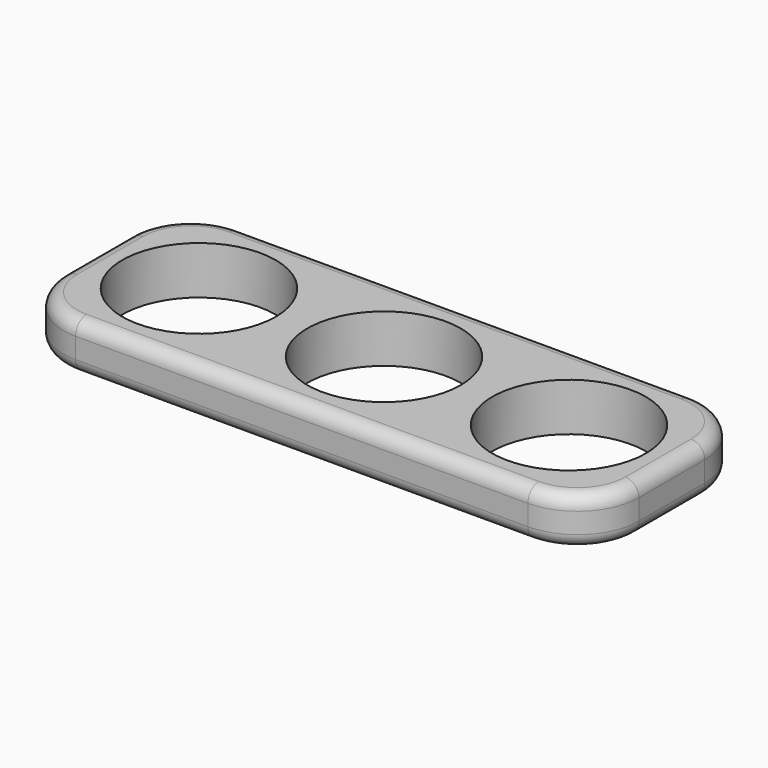
from build123d import *

# Parameters (mm, degrees)
F0_R         = 11.2
F1_DEPTH     = 7
F2_R         = 2
F3_T1_DEPTH  = 7
F3_T4_ANGLE  = 90
F3_T6_ANGLE  = 90
F3_T8_ANGLE  = 90
F3_T10_ANGLE = 90
F3_T12_ANGLE = 90
F3_T14_ANGLE = 90
F3_T16_ANGLE = 90
F3_T18_ANGLE = 90


# Not quite as in the source:
# - a fillet or chamfer that OpenCascade refuses, or shapes differently, is made with other operations: its cross-section is extruded or revolved along the edge and cut away or added


with BuildPart() as f1:
    # F0 (on Top) → F1 (new body)
    with BuildSketch(Plane.XY):
        Polygon((42, 15), (0, 15), (-42, 15), (-42, -15), (42, -15), align=None)
        with Locations((-27, 0)):
            Circle(F0_R, mode=Mode.SUBTRACT)
        Circle(F0_R, mode=Mode.SUBTRACT)
        with Locations((27, 0)):
            Circle(F0_R, mode=Mode.SUBTRACT)
    extrude(amount=F1_DEPTH)

    # F2
    f2_edges = [f1.edges().sort_by_distance(p)[0] for p in [
        (0, 15, 7),
        (-42, 0, 7),
        (0, -15, 7),
        (42, 0, 7),
        (42, 0, 0),
        (0, 15, 0),
        (-42, 0, 0),
        (0, -15, 0),
    ]]
    fillet(f2_edges, radius=F2_R)

    # F3: fillet of radius 9 on 4 edges, made by hand

    # F3_s2 → F3_t1 (cut)
    with BuildSketch(Plane.XY):
        with BuildLine():
            ThreePointArc((-33, 15), (-39.3639610307, 12.3639610307), (-42, 6))
            Line((-42, 6), (-42, 15))
            Line((-42, 15), (-33, 15))
        make_face()
        with BuildLine():
            ThreePointArc((-42, -6), (-39.3639610307, -12.3639610307), (-33, -15))
            Line((-33, -15), (-42, -15))
            Line((-42, -15), (-42, -6))
        make_face()
        with BuildLine():
            ThreePointArc((42, -6), (39.3639610307, -12.3639610307), (33, -15))
            Line((33, -15), (42, -15))
            Line((42, -15), (42, -6))
        make_face()
        with BuildLine():
            ThreePointArc((33, 15), (39.3639610307, 12.3639610307), (42, 6))
            Line((42, 6), (42, 15))
            Line((42, 15), (33, 15))
        make_face()
    extrude(amount=F3_T1_DEPTH, mode=Mode.SUBTRACT)

    # F3_s3 → F3_t4 (revolve, cut)
    with BuildSketch(Plane.YZ.offset(33)):
        with BuildLine():
            ThreePointArc((13, 0), (14.4142135624, 0.5857864376), (15, 2))
            Line((15, 2), (15, 0))
            Line((15, 0), (13, 0))
        make_face()
    revolve(axis=Axis((33, 6, 0), (0, 0, -1)), revolution_arc=F3_T4_ANGLE, mode=Mode.SUBTRACT)

    # F3_s5 → F3_t6 (revolve, cut)
    with BuildSketch(Plane.XZ.offset(-6)):
        with BuildLine():
            ThreePointArc((40, 7), (41.4142135624, 6.4142135624), (42, 5))
            Line((42, 5), (42, 7))
            Line((42, 7), (40, 7))
        make_face()
    revolve(axis=Axis((33, 6, 7), (0, 0, 1)), revolution_arc=F3_T6_ANGLE, mode=Mode.SUBTRACT)

    # F3_s7 → F3_t8 (revolve, cut)
    with BuildSketch(Plane.XZ.offset(6)):
        with BuildLine():
            ThreePointArc((40, 0), (41.4142135624, 0.5857864376), (42, 2))
            Line((42, 2), (42, 0))
            Line((42, 0), (40, 0))
        make_face()
    revolve(axis=Axis((33, -6, 0), (0, 0, -1)), revolution_arc=F3_T8_ANGLE, mode=Mode.SUBTRACT)

    # F3_s9 → F3_t10 (revolve, cut)
    with BuildSketch(Plane.YZ.offset(33)):
        with BuildLine():
            ThreePointArc((-13, 7), (-14.4142135624, 6.4142135624), (-15, 5))
            Line((-15, 5), (-15, 7))
            Line((-15, 7), (-13, 7))
        make_face()
    revolve(axis=Axis((33, -6, 7), (0, 0, 1)), revolution_arc=F3_T10_ANGLE, mode=Mode.SUBTRACT)

    # F3_s11 → F3_t12 (revolve, cut)
    with BuildSketch(Plane.YZ.offset(-33)):
        with BuildLine():
            ThreePointArc((-13, 0), (-14.4142135624, 0.5857864376), (-15, 2))
            Line((-15, 2), (-15, 0))
            Line((-15, 0), (-13, 0))
        make_face()
    revolve(axis=Axis((-33, -6, 0), (0, 0, -1)), revolution_arc=F3_T12_ANGLE, mode=Mode.SUBTRACT)

    # F3_s13 → F3_t14 (revolve, cut)
    with BuildSketch(Plane.XZ.offset(6)):
        with BuildLine():
            ThreePointArc((-40, 7), (-41.4142135624, 6.4142135624), (-42, 5))
            Line((-42, 5), (-42, 7))
            Line((-42, 7), (-40, 7))
        make_face()
    revolve(axis=Axis((-33, -6, 7), (0, 0, 1)), revolution_arc=F3_T14_ANGLE, mode=Mode.SUBTRACT)

    # F3_s15 → F3_t16 (revolve, cut)
    with BuildSketch(Plane.XZ.offset(-6)):
        with BuildLine():
            ThreePointArc((-40, 0), (-41.4142135624, 0.5857864376), (-42, 2))
            Line((-42, 2), (-42, 0))
            Line((-42, 0), (-40, 0))
        make_face()
    revolve(axis=Axis((-33, 6, 0), (0, 0, -1)), revolution_arc=F3_T16_ANGLE, mode=Mode.SUBTRACT)

    # F3_s17 → F3_t18 (revolve, cut)
    with BuildSketch(Plane.YZ.offset(-33)):
        with BuildLine():
            ThreePointArc((13, 7), (14.4142135624, 6.4142135624), (15, 5))
            Line((15, 5), (15, 7))
            Line((15, 7), (13, 7))
        make_face()
    revolve(axis=Axis((-33, 6, 7), (0, 0, 1)), revolution_arc=F3_T18_ANGLE, mode=Mode.SUBTRACT)


solid = f1.part
